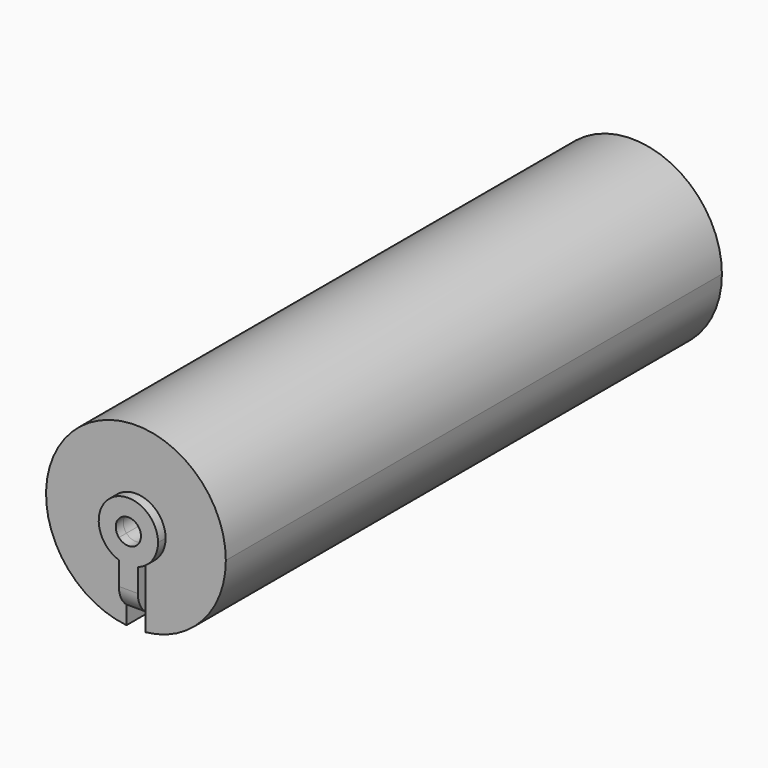
from build123d import *

# Parameters (mm, degrees)
F1_DEPTH    = 49.15
F2_DEPTH    = 0.75
F3_T1_DEPTH = 9.306247498
F4_R        = 2


# Not quite as in the source:
# - a fillet or chamfer that OpenCascade refuses, or shapes differently, is made with other operations: its cross-section is extruded or revolved along the edge and cut away or added


with BuildPart() as f1:
    # F0 (on Front) → F1 (new body)
    with BuildSketch(Plane.XZ):
        with BuildLine():
            ThreePointArc((0.75, -7.0854163604), (5.2966675844, -4.7655993852), (7.125, 0))
            ThreePointArc((7.125, 0), (-4.7655993852, 5.2966675844), (-0.75, -7.0854163604))
            Line((-0.75, -7.0854163604), (-0.75, -5.6354163604))
            Line((-0.75, -5.6354163604), (-0.75, -2.2271057451))
            ThreePointArc((-0.75, -2.2271057451), (-1.3711309201, 1.9085334684), (2.35, 0))
            ThreePointArc((2.35, 0), (1.9085334684, -1.3711309201), (0.75, -2.2271057451))
            Line((0.75, -2.2271057451), (0.75, -5.6354163604))
            Line((0.75, -5.6354163604), (0.75, -7.0854163604))
        make_face()
        with BuildLine():
            Line((-0.75, -2.2271057451), (-0.75, -5.6354163604))
            Line((-0.75, -5.6354163604), (0.75, -5.6354163604))
            Line((0.75, -5.6354163604), (0.75, -2.2271057451))
            ThreePointArc((0.75, -2.2271057451), (0, -2.35), (-0.75, -2.2271057451))
        make_face()
        with BuildLine():
            ThreePointArc((2.35, 0), (-1.3711309201, 1.9085334684), (-0.75, -2.2271057451))
            Line((-0.75, -2.2271057451), (-0.75, -0.6614378278))
            ThreePointArc((-0.75, -0.6614378278), (-0.3535533906, 0.9354143467), (1, 0))
            ThreePointArc((1, 0), (0.9354143467, -0.3535533906), (0.75, -0.6614378278))
            Line((0.75, -0.6614378278), (0.75, -2.2271057451))
            ThreePointArc((0.75, -2.2271057451), (1.9085334684, -1.3711309201), (2.35, 0))
        make_face()
        with BuildLine():
            Line((-0.75, -0.6614378278), (-0.75, -2.2271057451))
            ThreePointArc((-0.75, -2.2271057451), (0, -2.35), (0.75, -2.2271057451))
            Line((0.75, -2.2271057451), (0.75, -0.6614378278))
            ThreePointArc((0.75, -0.6614378278), (0, -1), (-0.75, -0.6614378278))
        make_face()
    extrude(amount=-F1_DEPTH)

    # F4
    f4_edges = [f1.edges().sort_by_distance(p)[0] for p in [
        (0, 49.15, -5.635416),
    ]]
    fillet(f4_edges, radius=F4_R)


with BuildPart() as f2:
    # F0 (on Front) → F2 (new body)
    with BuildSketch(Plane.XZ):
        with BuildLine():
            ThreePointArc((2.35, 0), (-1.3711309201, 1.9085334684), (-0.75, -2.2271057451))
            Line((-0.75, -2.2271057451), (-0.75, -0.6614378278))
            ThreePointArc((-0.75, -0.6614378278), (-0.3535533906, 0.9354143467), (1, 0))
            ThreePointArc((1, 0), (0.9354143467, -0.3535533906), (0.75, -0.6614378278))
            Line((0.75, -0.6614378278), (0.75, -2.2271057451))
            ThreePointArc((0.75, -2.2271057451), (1.9085334684, -1.3711309201), (2.35, 0))
        make_face()
        with BuildLine():
            Line((-0.75, -0.6614378278), (-0.75, -2.2271057451))
            ThreePointArc((-0.75, -2.2271057451), (0, -2.35), (0.75, -2.2271057451))
            Line((0.75, -2.2271057451), (0.75, -0.6614378278))
            ThreePointArc((0.75, -0.6614378278), (0, -1), (-0.75, -0.6614378278))
        make_face()
        with BuildLine():
            Line((-0.75, -2.2271057451), (-0.75, -5.6354163604))
            Line((-0.75, -5.6354163604), (0.75, -5.6354163604))
            Line((0.75, -5.6354163604), (0.75, -2.2271057451))
            ThreePointArc((0.75, -2.2271057451), (0, -2.35), (-0.75, -2.2271057451))
        make_face()
    extrude(amount=F2_DEPTH)

    # F3: fillet of radius 2 on 1 edges, made by hand

    # F3_s2 → F3_t1 (cut)
    with BuildSketch(Plane.YZ.offset(-4.653123749)):
        with BuildLine():
            ThreePointArc((0, -5.6354163604), (-0.5527756377, -4.9401922646), (-0.75, -4.0741668608))
            Line((-0.75, -4.0741668608), (-0.75, -5.6354163604))
            Line((-0.75, -5.6354163604), (0, -5.6354163604))
        make_face()
    extrude(amount=F3_T1_DEPTH, mode=Mode.SUBTRACT)


solid = Compound([f1.part, f2.part])
